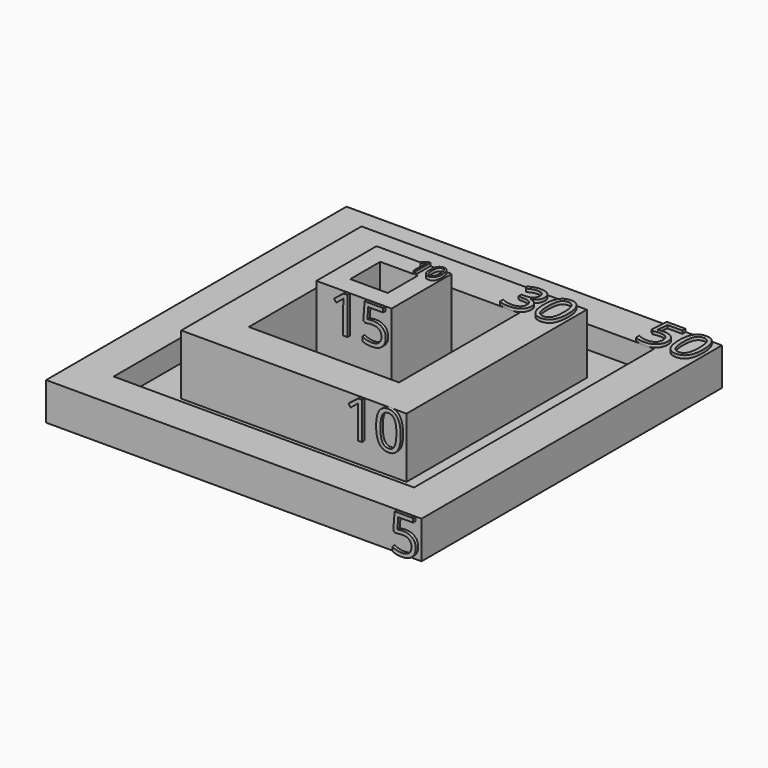
from build123d import *

# Parameters (mm, degrees)
F0_W          = 50
F0_H          = 50
F0_W_2        = 40
F0_H_2        = 40
F0_W_3        = 30
F0_H_3        = 30
F0_W_4        = 20
F0_H_4        = 20
F0_W_5        = 10
F0_H_5        = 10
F0_W_6        = 5
F0_H_6        = 5
F1_DEPTH      = 2
F2_DEPTH      = 3
F3_DEPTH      = 5
F4_DEPTH      = 10
F8_TEXT_SIZE  = 6.9444444444
F9_TEXT_SIZE  = 6.9444444444
F10_TEXT_SIZE = 3.4722222222
F11_DEPTH     = 0.4
F5_TEXT_SIZE  = 6.9444444444
F6_TEXT_SIZE  = 6.9490585288
F7_TEXT_SIZE  = 6.9352293781
F12_DEPTH     = 0.4


# Not quite as in the source:
# - Text() gives the source's letters only with a copy of the font that has no kerning and outlines rounded to 1/6400 em; it was checked with that copy


with BuildPart() as f1:
    # F0 (on Top) → F1 (new body)
    with BuildSketch(Plane.XY):
        Rectangle(F0_W, F0_H)
        Rectangle(F0_W_2, F0_H_2, mode=Mode.SUBTRACT)
        Rectangle(F0_W_2, F0_H_2)
        Rectangle(F0_W_3, F0_H_3, mode=Mode.SUBTRACT)
        Rectangle(F0_W_3, F0_H_3)
        Rectangle(F0_W_4, F0_H_4, mode=Mode.SUBTRACT)
        Rectangle(F0_W_4, F0_H_4)
        Rectangle(F0_W_5, F0_H_5, mode=Mode.SUBTRACT)
        Rectangle(F0_W_5, F0_H_5)
        Rectangle(F0_W_6, F0_H_6, mode=Mode.SUBTRACT)
        Rectangle(F0_W_6, F0_H_6)
    extrude(amount=-F1_DEPTH)

    # F0 (on Top) → F2 (join)
    with BuildSketch(Plane.XY):
        Rectangle(F0_W, F0_H)
        Rectangle(F0_W_2, F0_H_2, mode=Mode.SUBTRACT)
        Rectangle(F0_W_3, F0_H_3)
        Rectangle(F0_W_4, F0_H_4, mode=Mode.SUBTRACT)
        Rectangle(F0_W_5, F0_H_5)
        Rectangle(F0_W_6, F0_H_6, mode=Mode.SUBTRACT)
    extrude(amount=F2_DEPTH)

    # F3 (add): a face of the model
    f3_faces = [f1.faces().sort_by_distance(p)[0] for p in [
        (14.5757359313, 0, 3),
    ]]
    extrude(f3_faces, amount=F3_DEPTH)

    # F4 (add): a face of the model
    f4_faces = [f1.faces().sort_by_distance(p)[0] for p in [
        (4.8585786438, 0, 3),
    ]]
    extrude(f4_faces, amount=F4_DEPTH)

    # F8 (on face) + F9 (on face) + F10 (on face) → F11 (join)
    with BuildSketch(Plane.XY.offset(3)):
        with Locations((16.9542100694, 20)):
            Text('50', F8_TEXT_SIZE, font='Open Sans', text_align=(TextAlign.LEFT, TextAlign.BOTTOM))
    with BuildSketch(Plane.XY.offset(8)):
        with Locations((6.9542100694, 10)):
            Text('30', F9_TEXT_SIZE, font='Open Sans', text_align=(TextAlign.LEFT, TextAlign.BOTTOM))
    with BuildSketch(Plane.XY.offset(13)):
        with Locations((0.9771050347, 2.5)):
            Text('10', F10_TEXT_SIZE, font='Open Sans', text_align=(TextAlign.LEFT, TextAlign.BOTTOM))
    extrude(amount=F11_DEPTH)

    # F5 (on face) + F6 (on face) + F7 (on face) → F12 (join)
    with BuildSketch(Plane.XZ.offset(25)):
        with Locations((20.9787326389, -2)):
            Text('5', F5_TEXT_SIZE, font='Open Sans', text_align=(TextAlign.LEFT, TextAlign.BOTTOM))
    with BuildSketch(Plane.XZ.offset(15)):
        with Locations((6.9488642202, 2.9966778593)):
            Text('10', F6_TEXT_SIZE, font='Open Sans', text_align=(TextAlign.LEFT, TextAlign.BOTTOM))
    with BuildSketch(Plane.XZ.offset(5)):
        with Locations((-2.9809319328, 8.0066348477)):
            Text('15', F7_TEXT_SIZE, font='Open Sans', text_align=(TextAlign.LEFT, TextAlign.BOTTOM))
    extrude(amount=F12_DEPTH)


solid = f1.part
